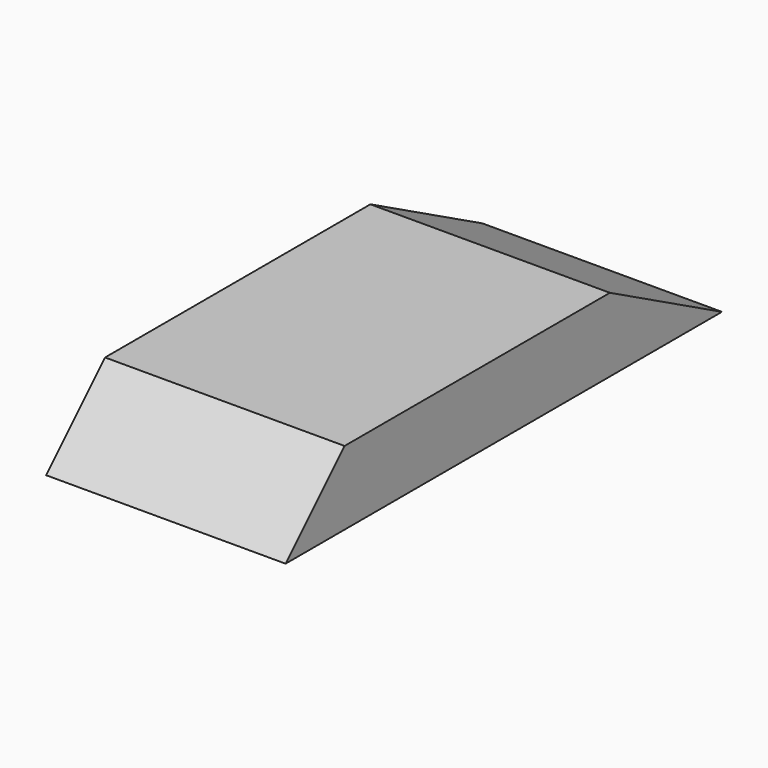
from build123d import *

# Parameters (mm, degrees)
F0_W     = 130
F0_H     = 296
F1_DEPTH = 20
F2_SIZE2 = 75.99999
F2_SIZE  = 39.99999
F3_SIZE2 = 39.99999
F3_SIZE  = 39.99999
F4_T     = 2.5


# Not quite as in the source:
# - a fillet or chamfer is up to 0.001 mm smaller than in the source, because OpenCascade refuses the exact size
# - a shell that OpenCascade refuses in one call is made with other operations: the cavity is built on its own and cut out


with BuildPart() as f1:
    # F0 (on Top) → F1 (new body, symmetric)
    with BuildSketch(Plane.XY):
        Rectangle(F0_W, F0_H)
    extrude(amount=F1_DEPTH, both=True)

    # F2 (size 40 and 76 in the source; OpenCascade refuses exactly that, so slightly less here)
    f2_edges = [f1.edges().sort_by_distance(p)[0] for p in [
        (0, 148, 20),
    ]]
    f2_side = f1.faces().sort_by_distance((0, 148, 0))[0]
    chamfer(f2_edges, length=F2_SIZE, length2=F2_SIZE2, reference=f2_side)

    # F3 (size 40 and 40 in the source; OpenCascade refuses exactly that, so slightly less here)
    f3_edges = [f1.edges().sort_by_distance(p)[0] for p in [
        (0, -148, 20),
    ]]
    chamfer(f3_edges, length=F3_SIZE, length2=F3_SIZE2)

    # F4: shell of thickness 2.5, made by hand


with BuildPart() as f4_core1:
    # F4_t2: copy of F1
    add(f1.part)

    # the walls: a layer under each face that stays
    f4_faces = [f4_core1.faces().sort_by_distance(p)[0] for p in [
        (-65, 0, 0),
        (0, -18, 20),
        (0, -128.000005, 5e-06),
        (0, 110.000005, 5e-06),
        (0, -148, -19.999995),
        (0, 148, -19.999995),
        (65, 0, 0),
    ]]
    thicken(f4_faces, amount=-F4_T, mode=Mode.SUBTRACT)


with BuildPart() as f1_1:
    add(f1.part)

    # what is left inside the walls is the cavity
    f4_cavity = [f4_core1.part.solids().sort_by_distance(p)[0] for p in [
        (0, -48.765554, -19.975),
    ]]
    add(f4_cavity, mode=Mode.SUBTRACT)


solid = f1_1.part
